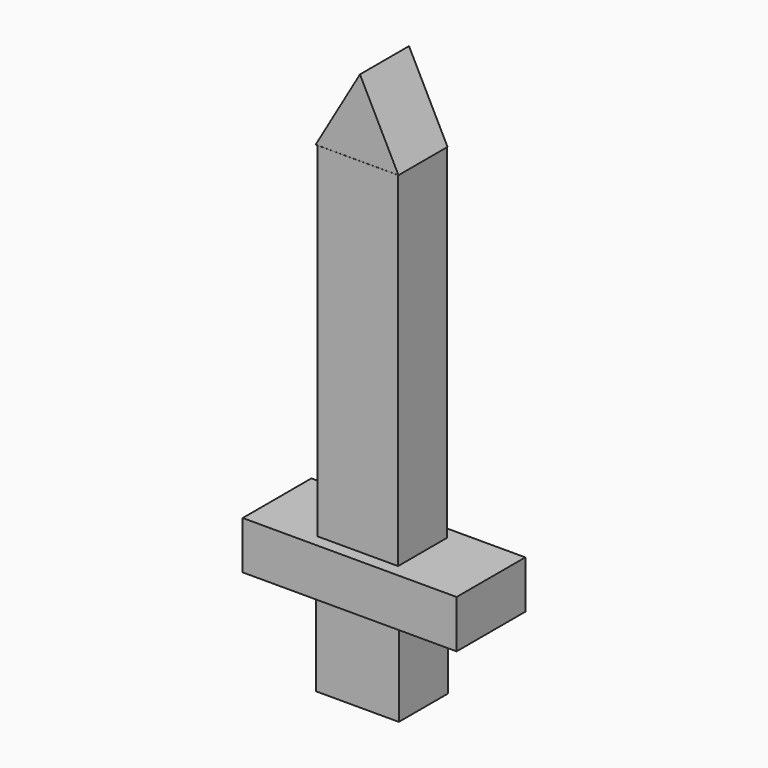
from build123d import *

# Parameters (mm, degrees)
F3_DEPTH = 10
F2_W     = 13.4988240898
F2_H     = 14.4473891705
F1_W     = 34.8780401982
F1_H     = 7.810738869
F4_DEPTH = 12
F5_DEPTH = 2
F6_W     = 13.1339915097
F6_H     = 56.1272315681
F7_DEPTH = 10


# Not quite as in the source:
# - a feature names something its author has since deleted; it is built from what else it names


with BuildPart() as f3:
    # F0 (on Front) → F3 (new body)
    with BuildSketch(Plane.XZ):
        Polygon((-23.6272681504, 68.5679614544), (-30.8464840055, 56.137226522), (-17.3418466002, 56.137226522), align=None)
    extrude(amount=F3_DEPTH)


with BuildPart() as f3b:
    # F2 (on Front) → F3, piece 2 (new body)
    with BuildSketch(Plane.XZ):
        with Locations((-24.0321997553, -15.107399784)):
            Rectangle(F2_W, F2_H)
    extrude(amount=F3_DEPTH)


with BuildPart() as f4:
    # F1 (on Front) → F4 (new body)
    with BuildSketch(Plane.XZ):
        with Locations((-23.7038496416, -3.9053694345)):
            Rectangle(F1_W, F1_H)
    extrude(amount=F4_DEPTH)

    # F5 (add): a face of the model
    f5_faces = [f4.faces().sort_by_distance(p)[0] for p in [
        (-23.7038496416, 0, -3.9053694345),
    ]]
    extrude(f5_faces, amount=F5_DEPTH)

    # F6 (on Front) → F7 (join)
    with BuildSketch(Plane.XZ):
        with Locations((-23.975726217, 28.063615784)):
            Rectangle(F6_W, F6_H)
    extrude(amount=F7_DEPTH)


solid = Compound([f3.part, f3b.part, f4.part])
